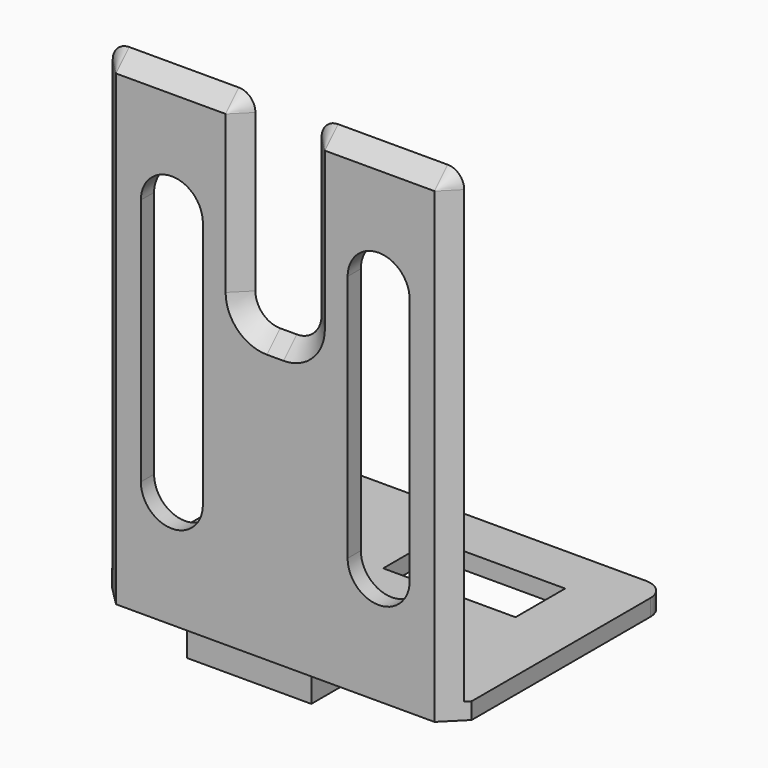
from build123d import *

# Parameters (mm, degrees)
F1_DEPTH      = 4
F2_W          = 87
F2_H          = 4
F3_DEPTH      = 60
F4_W          = 32
F4_H          = 15
F5_DEPTH      = 4
F6_R          = 5
F7_W          = 30
F7_H          = 30
F7_R          = 2.75
F8_DEPTH      = 9
F9_DEPTH      = 5
F10_T1_DEPTH  = 26.5
F10_T3_DEPTH  = 125.8584149398
F10_T5_DEPTH  = 38
F10_T7_DEPTH  = 4
F10_T9_DEPTH  = 26.5
F10_T12_ANGLE = 90
F10_T14_ANGLE = 90
F10_T16_ANGLE = 90
F10_T18_ANGLE = 90
F10_T20_ANGLE = 90
F10_T22_ANGLE = 90
F11_W         = 11.3
F11_H         = 5.2
F12_DEPTH     = 30.7


# Not quite as in the source:
# - a fillet or chamfer that OpenCascade refuses, or shapes differently, is made with other operations: its cross-section is extruded or revolved along the edge and cut away or added


with BuildPart() as f1:
    # F0 (on Front) → F1 (new body)
    with BuildSketch(Plane.XZ):
        Polygon((-7, 78.3899563551), (-43.5, 78.3899563551), (-43.5, -39.6100436449), (43.5, -39.6100436449), (43.5, 78.3899563551), (7, 78.3899563551), (7, 30.3899563551), (-7, 30.3899563551), align=None)
        with BuildLine():
            Line((-17.5, 48.3899563551), (-17.5, -11.6100436449))
            ThreePointArc((-17.5, -11.6100436449), (-25, -19.1100436449), (-32.5, -11.6100436449))
            Line((-32.5, -11.6100436449), (-32.5, 48.3899563551))
            ThreePointArc((-32.5, 48.3899563551), (-25, 55.8899563551), (-17.5, 48.3899563551))
        make_face(mode=Mode.SUBTRACT)
        with BuildLine():
            Line((32.5, 48.3899563551), (32.5, -11.6100436449))
            ThreePointArc((32.5, -11.6100436449), (25, -19.1100436449), (17.5, -11.6100436449))
            Line((17.5, -11.6100436449), (17.5, 48.3899563551))
            ThreePointArc((17.5, 48.3899563551), (25, 55.8899563551), (32.5, 48.3899563551))
        make_face(mode=Mode.SUBTRACT)
    extrude(amount=F1_DEPTH)

    # F2 (on face) → F3 (join)
    with BuildSketch(Plane(origin=(0, 0, 0), x_dir=(-1, 0, 0), z_dir=(0, 1, 0))):
        with Locations((0, -37.6100436449)):
            Rectangle(F2_W, F2_H)
    extrude(amount=F3_DEPTH)

    # F4 (on face) → F5 (cut)
    with BuildSketch(Plane(origin=(0, 0, -39.6100436449), x_dir=(1, 0, 0), z_dir=(0, 0, -1))):
        with Locations((12.5, -40.5)):
            Rectangle(F4_W, F4_H)
    extrude(amount=-F5_DEPTH, mode=Mode.SUBTRACT)

    # F6
    f6_edges = [f1.edges().sort_by_distance(p)[0] for p in [
        (-43.5, -2, 78.389956),
        (7, -2, 78.389956),
        (-7, -2, 78.389956),
        (43.5, -2, 78.389956),
        (-43.5, 60, -37.610044),
        (43.5, 60, -37.610044),
        (7, -2, 30.389956),
        (-7, -2, 30.389956),
    ]]
    fillet(f6_edges, radius=F6_R)

    # F7 (on face) → F8 (join)
    with BuildSketch(Plane(origin=(0, 0, -39.6100436449), x_dir=(1, 0, 0), z_dir=(0, 0, -1))):
        with Locations((-10.0618535653, -15.7216744063)):
            Rectangle(F7_W, F7_H)
        with Locations((-10.0618535653, -15.7216744063)):
            Circle(F7_R, mode=Mode.SUBTRACT)
    extrude(amount=F8_DEPTH)

    # F9 (cut): a face of the model
    f9_faces = [f1.faces().sort_by_distance(p)[0] for p in [
        (-10.0618535653, 15.7216744063, -39.6100436449),
    ]]
    extrude(f9_faces, amount=-F9_DEPTH, mode=Mode.SUBTRACT)

    # F10: chamfer of 5 on 1 edges, made by hand

    # F10_s2 → F10_t1 (cut)
    with BuildSketch(Plane.YZ.offset(-38.5)):
        Polygon((-4, 73.3899563551), (1, 78.3899563551), (-4, 78.3899563551), align=None)
    extrude(amount=F10_T1_DEPTH, mode=Mode.SUBTRACT)

    # F10_s4 → F10_t3 (cut)
    with BuildSketch(Plane.XY.offset(-52.4684585847)):
        Polygon((-38.5, -4), (-43.5, 1), (-43.5, -4), align=None)
        Polygon((38.5, -4), (43.5, 1), (43.5, -4), align=None)
    extrude(amount=F10_T3_DEPTH, mode=Mode.SUBTRACT)

    # F10_s6 → F10_t5 (cut)
    with BuildSketch(Plane.XY.offset(35.3899563551)):
        Polygon((-7, 1), (-12, -4), (-7, -4), align=None)
        Polygon((12, -4), (7, 1), (7, -4), align=None)
    extrude(amount=F10_T5_DEPTH, mode=Mode.SUBTRACT)

    # F10_s8 → F10_t7 (cut)
    with BuildSketch(Plane.YZ.offset(-2)):
        Polygon((-4, 25.3899563551), (1, 30.3899563551), (-4, 30.3899563551), align=None)
    extrude(amount=F10_T7_DEPTH, mode=Mode.SUBTRACT)

    # F10_s10 → F10_t9 (cut)
    with BuildSketch(Plane.YZ.offset(12)):
        Polygon((-4, 73.3899563551), (1, 78.3899563551), (-4, 78.3899563551), align=None)
    extrude(amount=F10_T9_DEPTH, mode=Mode.SUBTRACT)

    # F10_s11 → F10_t12 (revolve, cut)
    with BuildSketch(Plane.XY.offset(73.3899563551)):
        Polygon((-7, 1), (-12, -4), (-7, -4), align=None)
    revolve(axis=Axis((-12, -4, 73.3899563551), (0, -1, 0)), revolution_arc=F10_T12_ANGLE, mode=Mode.SUBTRACT)

    # F10_s13 → F10_t14 (revolve, cut)
    with BuildSketch(Plane.YZ.offset(-38.5)):
        Polygon((-4, 73.3899563551), (1, 78.3899563551), (-4, 78.3899563551), align=None)
    revolve(axis=Axis((-38.5, -4, 73.3899563551), (0, -1, 0)), revolution_arc=F10_T14_ANGLE, mode=Mode.SUBTRACT)

    # F10_s15 → F10_t16 (revolve, cut)
    with BuildSketch(Plane.XY.offset(35.3899563551)):
        Polygon((-7, 1), (-12, -4), (-7, -4), align=None)
    revolve(axis=Axis((-2, -4, 35.3899563551), (0, -1, 0)), revolution_arc=F10_T16_ANGLE, mode=Mode.SUBTRACT)

    # F10_s17 → F10_t18 (revolve, cut)
    with BuildSketch(Plane.YZ.offset(2)):
        Polygon((-4, 25.3899563551), (1, 30.3899563551), (-4, 30.3899563551), align=None)
    revolve(axis=Axis((2, -4, 35.3899563551), (0, -1, 0)), revolution_arc=F10_T18_ANGLE, mode=Mode.SUBTRACT)

    # F10_s19 → F10_t20 (revolve, cut)
    with BuildSketch(Plane.XY.offset(73.3899563551)):
        Polygon((12, -4), (7, 1), (7, -4), align=None)
    revolve(axis=Axis((12, -4, 73.3899563551), (0, 1, 0)), revolution_arc=F10_T20_ANGLE, mode=Mode.SUBTRACT)

    # F10_s21 → F10_t22 (revolve, cut)
    with BuildSketch(Plane.YZ.offset(38.5)):
        Polygon((-4, 73.3899563551), (1, 78.3899563551), (-4, 78.3899563551), align=None)
    revolve(axis=Axis((38.5, -4, 73.3899563551), (0, 1, 0)), revolution_arc=F10_T22_ANGLE, mode=Mode.SUBTRACT)

    # F11 (on face) → F12 (cut)
    with BuildSketch(Plane.YZ.offset(4.9381464347)):
        with Locations((16.5075063076, -44.0100436449)):
            Rectangle(F11_W, F11_H)
    extrude(amount=-F12_DEPTH, mode=Mode.SUBTRACT)


solid = f1.part
